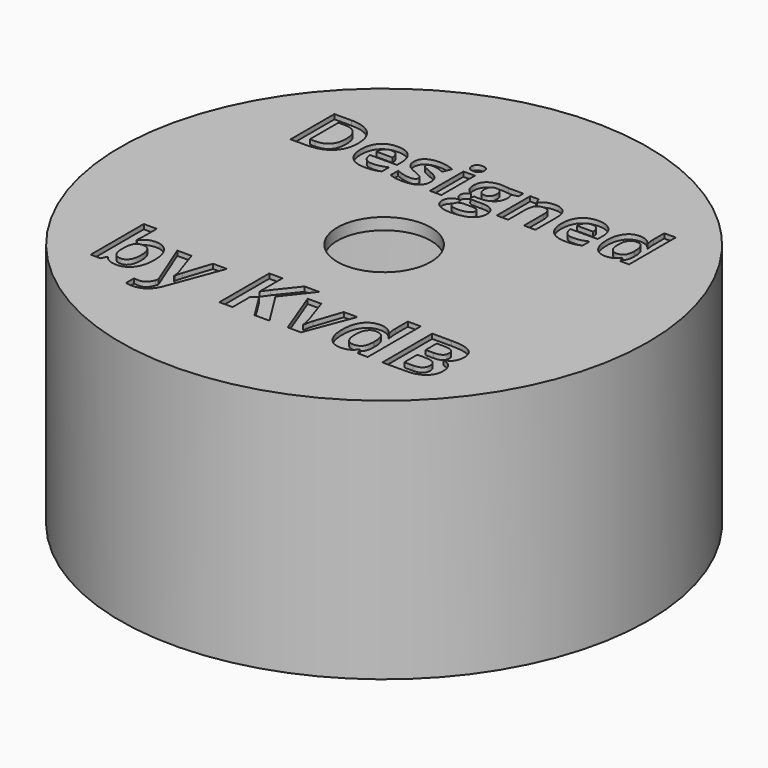
from build123d import *

# Parameters (mm, degrees)
F0_R           = 113
F0_R_2         = 110
F1_DEPTH       = 100
F2_R           = 113
F2_R_2         = 110
F2_R_3         = 20
F3_DEPTH       = 5
F4_TEXT_SIZE   = 32.849712565
F4_TEXT_SIZE_2 = 37.393370467
F5_DEPTH       = 2


# Not quite as in the source:
# - Text() gives the source's letters only with a copy of the font that has no kerning and outlines rounded to 1/6400 em; it was checked with that copy


with BuildPart() as f1:
    # F0 (on Top) → F1 (new body)
    with BuildSketch(Plane.XY):
        Circle(F0_R)
        Circle(F0_R_2, mode=Mode.SUBTRACT)
    extrude(amount=F1_DEPTH)

    # F2 (on face) → F3 (join)
    with BuildSketch(Plane.XY.offset(100)):
        Circle(F2_R)
        Circle(F2_R_2, mode=Mode.SUBTRACT)
        Circle(F2_R_2)
        Circle(F2_R_3, mode=Mode.SUBTRACT)
    extrude(amount=F3_DEPTH)

    # F4 (on face) → F5 (cut)
    with BuildSketch(Plane.XY.offset(105)):
        with Locations((-75, 40)):
            Text('Designed', F4_TEXT_SIZE, font='Open Sans', font_style=FontStyle.BOLD, text_align=(TextAlign.LEFT, TextAlign.BOTTOM))
        with Locations((-75, -66.9232267363)):
            Text('by KvdB', F4_TEXT_SIZE_2, font='Open Sans', font_style=FontStyle.BOLD, text_align=(TextAlign.LEFT, TextAlign.BOTTOM))
    extrude(amount=-F5_DEPTH, mode=Mode.SUBTRACT)


solid = f1.part
